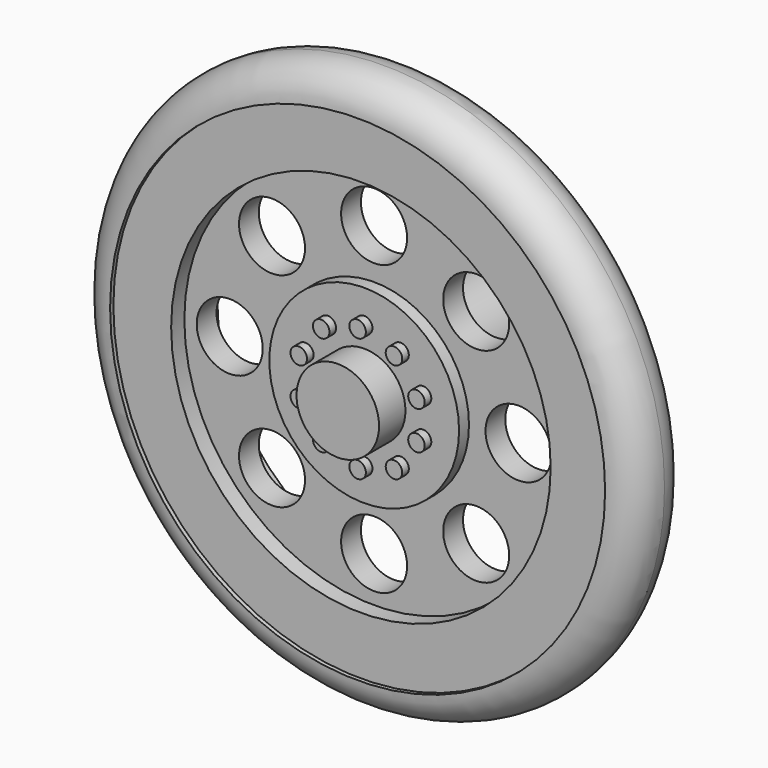
from build123d import *

# Parameters (mm, degrees)
F0_R      = 17
F1_DEPTH  = 4
F2_R      = 2
F3_R      = 1.99999
F4_R      = 15
F4_R_2    = 2
F4_R_3    = 5.75
F5_DEPTH  = 0.25
F6_DEPTH  = 0.25
F7_R      = 11.5
F7_R_2    = 2
F7_R_3    = 5.75
F8_DEPTH  = 1
F9_R      = 11.5
F10_DEPTH = 1
F11_DEPTH = 5
F12_DEPTH = 0.5
F13_R     = 0.5
F14_DEPTH = 0.5
F13_R_2   = 2.5
F15_DEPTH = 2
F16_R     = 3
F17_DEPTH = 8.5
F18_R     = 1.5
F19_DEPTH = 9


# Not quite as in the source:
# - a fillet or chamfer is up to 0.001 mm smaller than in the source, because OpenCascade refuses the exact size


with BuildPart() as f1:
    # F0 (on Front) → F1 (new body)
    with BuildSketch(Plane.XZ):
        Circle(F0_R)
    extrude(amount=-F1_DEPTH)

    # F2
    f2_edges = [f1.edges().sort_by_distance(p)[0] for p in [
        (-17, 0, 0),
    ]]
    fillet(f2_edges, radius=F2_R)

    # F3 (radius 2 in the source; OpenCascade refuses exactly that, so slightly less here)
    f3_edges = [f1.edges().sort_by_distance(p)[0] for p in [
        (-17, 4, 0),
    ]]
    fillet(f3_edges, radius=F3_R)

    # F4 (on face) → F5 (cut)
    with BuildSketch(Plane.XZ):
        Circle(F4_R)
        with Locations((-6.1871843354, -6.1871843354)):
            Circle(F4_R_2, mode=Mode.SUBTRACT)
        with Locations((0, -8.75)):
            Circle(F4_R_2, mode=Mode.SUBTRACT)
        with Locations((6.1871843354, -6.1871843354)):
            Circle(F4_R_2, mode=Mode.SUBTRACT)
        with Locations((-8.75, 0)):
            Circle(F4_R_2, mode=Mode.SUBTRACT)
        with Locations((-6.1871843354, 6.1871843354)):
            Circle(F4_R_2, mode=Mode.SUBTRACT)
        Circle(F4_R_3, mode=Mode.SUBTRACT)
        with Locations((6.1871843354, 6.1871843354)):
            Circle(F4_R_2, mode=Mode.SUBTRACT)
        with Locations((8.75, 0)):
            Circle(F4_R_2, mode=Mode.SUBTRACT)
        with Locations((0, 8.75)):
            Circle(F4_R_2, mode=Mode.SUBTRACT)
    extrude(amount=-F5_DEPTH, mode=Mode.SUBTRACT)

    # F6 (cut): a face of the model
    f6_faces = [f1.faces().sort_by_distance(p)[0] for p in [
        (0, 4, 0),
    ]]
    extrude(f6_faces, amount=-F6_DEPTH, mode=Mode.SUBTRACT)

    # F7 (on face) → F8 (cut)
    with BuildSketch(Plane.XZ.offset(-0.25)):
        Circle(F7_R)
        with Locations((-6.1871843354, -6.1871843354)):
            Circle(F7_R_2, mode=Mode.SUBTRACT)
        with Locations((0, -8.75)):
            Circle(F7_R_2, mode=Mode.SUBTRACT)
        with Locations((6.1871843354, -6.1871843354)):
            Circle(F7_R_2, mode=Mode.SUBTRACT)
        with Locations((-8.75, 0)):
            Circle(F7_R_2, mode=Mode.SUBTRACT)
        with Locations((-6.1871843354, 6.1871843354)):
            Circle(F7_R_2, mode=Mode.SUBTRACT)
        Circle(F7_R_3, mode=Mode.SUBTRACT)
        with Locations((6.1871843354, 6.1871843354)):
            Circle(F7_R_2, mode=Mode.SUBTRACT)
        with Locations((8.75, 0)):
            Circle(F7_R_2, mode=Mode.SUBTRACT)
        with Locations((0, 8.75)):
            Circle(F7_R_2, mode=Mode.SUBTRACT)
    extrude(amount=-F8_DEPTH, mode=Mode.SUBTRACT)

    # F9 (on face) → F10 (cut)
    with BuildSketch(Plane(origin=(0, 3.75, 0), x_dir=(-1, 0, 0), z_dir=(0, 1, 0))):
        Circle(F9_R)
    extrude(amount=-F10_DEPTH, mode=Mode.SUBTRACT)

    # F11 (cut): faces of the model
    f11_faces = [f1.faces().sort_by_distance(p)[0] for p in [
        (8.75, 0, 0),
        (6.1871843354, 0, -6.1871843354),
        (0, 0, -8.75),
        (-8.75, 0, 0),
        (0, 0, 8.75),
        (6.1871843354, 0, 6.1871843354),
        (-6.1871843354, 0, -6.1871843354),
        (-6.1871843354, 0, 6.1871843354),
    ]]
    extrude(f11_faces, amount=-F11_DEPTH, mode=Mode.SUBTRACT)

    # F12 (cut): a face of the model
    f12_faces = [f1.faces().sort_by_distance(p)[0] for p in [
        (0, 0, 0),
    ]]
    extrude(f12_faces, amount=-F12_DEPTH, mode=Mode.SUBTRACT)

    # F13 (on face) → F14 (join)
    with BuildSketch(Plane.XZ.offset(-0.5)):
        with Locations((-2.2041946961, 3.0338137289)):
            Circle(F13_R)
        with Locations((-3.5664619361, 1.1588137289)):
            Circle(F13_R)
        with Locations((-3.5664619361, -1.1588137289)):
            Circle(F13_R)
        with Locations((-2.2041946961, -3.0338137289)):
            Circle(F13_R)
        with Locations((2.2041946961, -3.0338137289)):
            Circle(F13_R)
        with Locations((3.5664619361, -1.1588137289)):
            Circle(F13_R)
        with Locations((3.5664619361, 1.1588137289)):
            Circle(F13_R)
        with Locations((2.2041946961, 3.0338137289)):
            Circle(F13_R)
        with Locations((0, 3.75)):
            Circle(F13_R)
        with Locations((0, -3.75)):
            Circle(F13_R)
    extrude(amount=F14_DEPTH)

    # F13 (on face) → F15 (join)
    with BuildSketch(Plane.XZ.offset(-0.5)):
        Circle(F13_R_2)
    extrude(amount=F15_DEPTH)

    # F16 (on face) → F17 (join)
    with BuildSketch(Plane(origin=(0, 2.75, 0), x_dir=(-1, 0, 0), z_dir=(0, 1, 0))):
        Circle(F16_R)
    extrude(amount=F17_DEPTH)

    # F18 (on face) → F19 (cut)
    with BuildSketch(Plane(origin=(0, 11.25, 0), x_dir=(-1, 0, 0), z_dir=(0, 1, 0))):
        Circle(F18_R)
    extrude(amount=-F19_DEPTH, mode=Mode.SUBTRACT)


solid = f1.part
